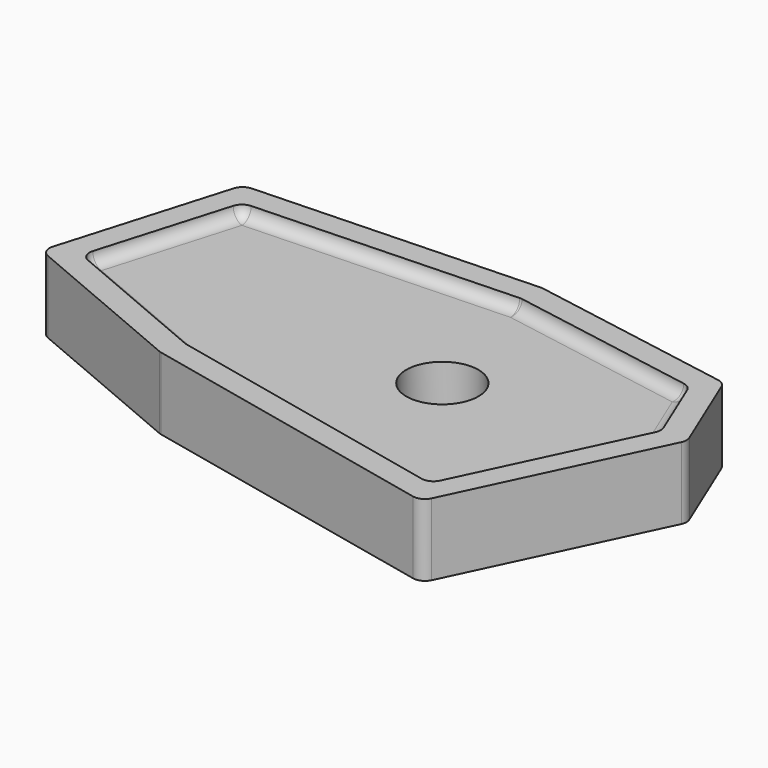
from build123d import *

# Parameters (mm, degrees)
F1_DEPTH = 15
F2_T     = -10
F3_R     = 4.99999
F5_R     = 15
F6_DEPTH = 25


# Not quite as in the source:
# - a fillet or chamfer is up to 0.001 mm smaller than in the source, because OpenCascade refuses the exact size


with BuildPart() as f1:
    # F0 (on Top) → F1 (new body)
    with BuildSketch(Plane.XY):
        Polygon((87.8512188792, -15.3126027435), (0, 0), (-120.9431961179, -4.3791108765), (-143.5155719519, -80.9135511518), (-68.7445923686, -112.6559451222), (62.802106142, -141.5623724461), (104.0751114488, -54.4615574181), align=None)
    extrude(amount=F1_DEPTH)

    # F2
    f2_openings = [f1.faces().sort_by_distance(p)[0] for p in [
        (-14.831711, -62.307507, 15),
    ]]
    offset(amount=F2_T, openings=f2_openings)

    # F3 (radius 5 in the source; OpenCascade refuses exactly that, so slightly less here)
    f3_edges = [f1.edges().sort_by_distance(p)[0] for p in [
        (-143.515572, -80.913551, 7.5),
        (-68.744592, -112.655945, 7.5),
        (62.802106, -141.562372, 7.5),
        (104.075111, -54.461557, 7.5),
        (87.851219, -15.312603, 7.5),
        (0, 0, 7.5),
        (-120.943196, -4.379111, 7.5),
        (75.155878, -92.138524, 10),
        (-4.258831, -116.587633, 10),
        (57.17386, -130.087018, 12.5),
        (-65.691523, -103.088247, 12.5),
        (-98.546913, -89.140205, 10),
        (86.927893, -39.205026, 10),
        (93.137896, -54.19003, 12.5),
        (80.717891, -24.220021, 12.5),
        (40.016406, -17.12569, 10),
        (-0.685079, -10.031358, 12.5),
        (-57.036491, -12.07173, 10),
        (-122.395103, -44.652133, 10),
        (-113.387903, -14.112102, 12.5),
        (-131.402304, -75.192163, 12.5),
    ]]
    fillet(f3_edges, radius=F3_R)

    # F4: F1 across plane


with BuildPart() as f1_1:
    add(f1.part)
    add(f1.part.mirror(Plane.XY))

    # F5 (on face) → F6 (cut)
    with BuildSketch(Plane.XY.offset(10)):
        with Locations((10.5543992388, -65)):
            Circle(F5_R)
    extrude(amount=-F6_DEPTH, mode=Mode.SUBTRACT)


solid = f1_1.part
